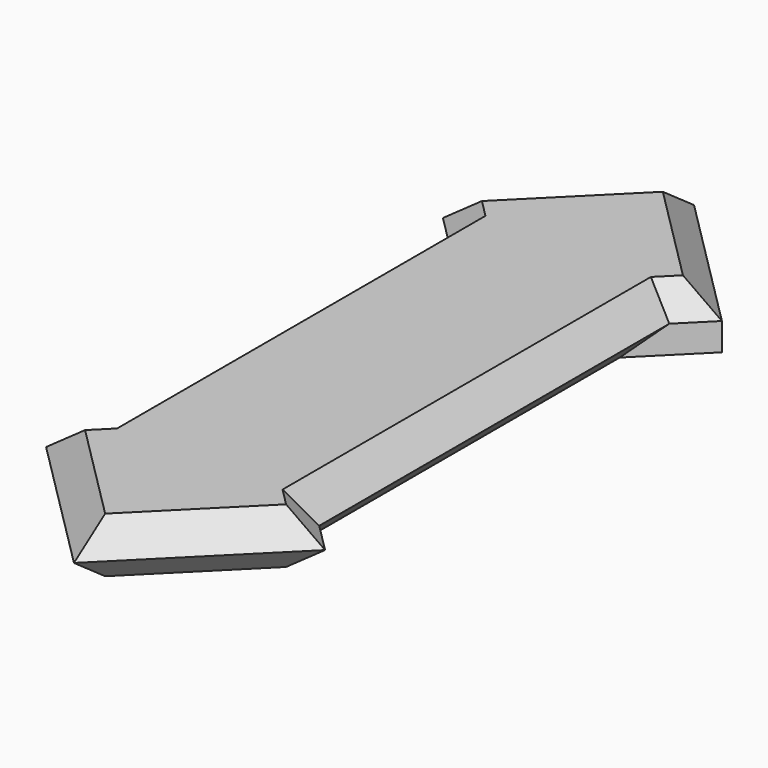
from build123d import *

# Parameters (mm, degrees)
F1_DEPTH = 20
F2_SIZE2 = 9.99999
F2_SIZE  = 9.99999


# Not quite as in the source:
# - a fillet or chamfer is up to 0.001 mm smaller than in the source, because OpenCascade refuses the exact size


with BuildPart() as f1:
    # F0 (on Top) → F1 (new body)
    with BuildSketch(Plane.XY):
        Polygon((-50.6066017178, 10.6066017178), (-40, 0), (-40, -79.367487377), (40, -79.367487377), (40, 0), (50.6066017178, 10.6066017178), (0, 61.2132034356), align=None)
        Polygon((40, -79.367487377), (-40, -79.367487377), (-40, -158.7349747541), (-50.6066017178, -169.3415764719), (0, -219.9481781897), (50.6066017178, -169.3415764719), (40, -158.7349747541), align=None)
    extrude(amount=F1_DEPTH)

    # F2 (size 10 and 10 in the source; OpenCascade refuses exactly that, so slightly less here)
    f2_edges = [f1.edges().sort_by_distance(p)[0] for p in [
        (40, -79.367487, 20),
        (25.303301, 35.909903, 20),
        (-25.303301, 35.909903, 20),
        (-45.303301, 5.303301, 20),
        (45.303301, 5.303301, 20),
        (-40, -79.367487, 20),
        (-45.303301, -164.038276, 20),
        (-25.303301, -194.644877, 20),
        (25.303301, -194.644877, 20),
        (45.303301, -164.038276, 20),
        (40, -79.367487, 0),
        (25.303301, -194.644877, 0),
        (45.303301, -164.038276, 0),
        (-25.303301, -194.644877, 0),
        (-45.303301, -164.038276, 0),
        (-40, -79.367487, 0),
        (-45.303301, 5.303301, 0),
        (-25.303301, 35.909903, 0),
    ]]
    chamfer(f2_edges, length=F2_SIZE, length2=F2_SIZE2)


solid = f1.part
